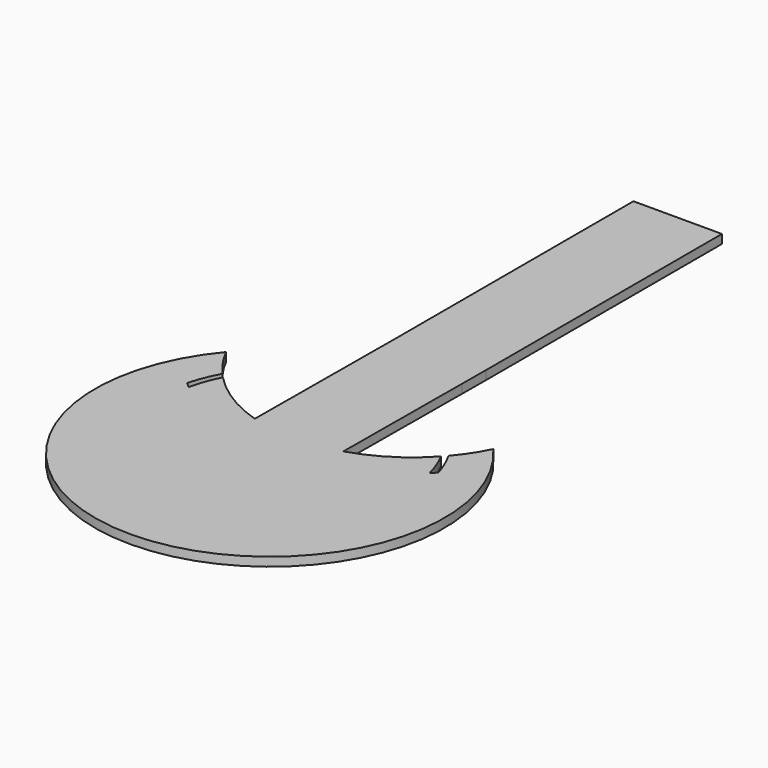
from build123d import *

# Parameters (mm, degrees)
F0_W     = 60
F0_H     = 200
F1_DEPTH = 6


# Not quite as in the source:
# - the program builds the solid bodies; features that only make, move or delete a surface that nothing else refers to are left out


with BuildPart() as f1:
    # F0 (on Top) → F1 (new body)
    with BuildSketch(Plane.XY):
        with Locations((4.8876879096, 35.2179194741)):
            Rectangle(F0_W, F0_H)
        with BuildLine():
            ThreePointArc((-79.4584430704, -175.2136584167), (-76.086405566, -164.9666401832), (-71.4764851469, -155.2136584167))
            ThreePointArc((-71.4764851469, -155.2136584167), (-79.1565485083, -145.3205641479), (-85.5490516624, -134.5505784994))
            ThreePointArc((-85.5490516624, -134.5505784994), (6.1468085688, -329.3233337338), (94.4628409087, -132.9949471034))
            ThreePointArc((94.4628409087, -132.9949471034), (88.2574232589, -143.8738017875), (80.7494829473, -153.8981481364))
            ThreePointArc((80.7494829473, -153.8981481364), (85.2254366965, -162.8589485125), (88.6456429035, -172.2734211397))
            ThreePointArc((88.6456429035, -172.2734211397), (75.2367314586, -249.2062042963), (5.6459887203, -284.6403764396))
            ThreePointArc((5.6459887203, -284.6403764396), (-63.9155377146, -250.9329661403), (-79.4584430704, -175.2136584167))
        make_face()
        with BuildLine():
            ThreePointArc((4.8876879096, -189.3289751767), (-10.6634233248, -188.2490297182), (-25.8614792361, -184.7816907769))
            ThreePointArc((-25.8614792361, -184.7816907769), (-48.9823809676, -174.2243385437), (-68.7229965841, -158.2136584167))
            ThreePointArc((-68.7229965841, -158.2136584167), (-72.9335538665, -167.9839691049), (-75.8560904631, -178.2136584167))
            ThreePointArc((-75.8560904631, -178.2136584167), (-59.2361153237, -247.9542245013), (5.5975931326, -278.5574984969))
            Line((5.5975931326, -278.5574984969), (4.8876879096, -189.3289751767))
        make_face()
        with BuildLine():
            ThreePointArc((78.0917461365, -156.8981481364), (57.9442467877, -173.7054474984), (34.1385207639, -184.7369682609))
            ThreePointArc((34.1385207639, -184.7369682609), (19.6828166371, -188.1140297879), (4.8876879096, -189.3289751767))
            Line((4.8876879096, -189.3289751767), (5.5975931326, -278.5574984969))
            ThreePointArc((5.5975931326, -278.5574984969), (70.4913174106, -246.4384867175), (85.2871903638, -175.5589515052))
            ThreePointArc((85.2871903638, -175.5589515052), (82.255170922, -166.010419768), (78.0917461365, -156.8981481364))
        make_face()
        with BuildLine():
            ThreePointArc((5.5975931326, -278.5574984969), (-59.2361153237, -247.9542245013), (-75.8560904631, -178.2136584167))
            Line((-75.8560904631, -178.2136584167), (-79.4584430704, -175.2136584167))
            ThreePointArc((-79.4584430704, -175.2136584167), (-63.9155377146, -250.9329661403), (5.6459887203, -284.6403764396))
            Line((5.6459887203, -284.6403764396), (5.5975931326, -278.5574984969))
        make_face()
        with BuildLine():
            ThreePointArc((85.2871903638, -175.5589515052), (70.4913174106, -246.4384867175), (5.5975931326, -278.5574984969))
            Line((5.5975931326, -278.5574984969), (5.6459887203, -284.6403764396))
            ThreePointArc((5.6459887203, -284.6403764396), (75.2367314586, -249.2062042963), (88.6456429035, -172.2734211397))
            Line((88.6456429035, -172.2734211397), (85.2871903638, -175.5589515052))
        make_face()
        with BuildLine():
            Line((34.7627821954, -84.7816907769), (-25.2371712536, -84.7816907769))
            Line((-25.2371712536, -84.7816907769), (-25.8614792361, -184.7816907769))
            ThreePointArc((-25.8614792361, -184.7816907769), (-10.6634233248, -188.2490297182), (4.8876879096, -189.3289751767))
            ThreePointArc((4.8876879096, -189.3289751767), (19.6828166371, -188.1140297879), (34.1385207639, -184.7369682609))
            Line((34.1385207639, -184.7369682609), (34.7627821954, -84.7816907769))
        make_face()
        Polygon((34.8876879096, -64.7820805259), (-25.1123120904, -64.7820805259), (-25.2371712536, -84.7816907769), (34.7627821954, -84.7816907769), align=None)
    extrude(amount=F1_DEPTH)


solid = f1.part
